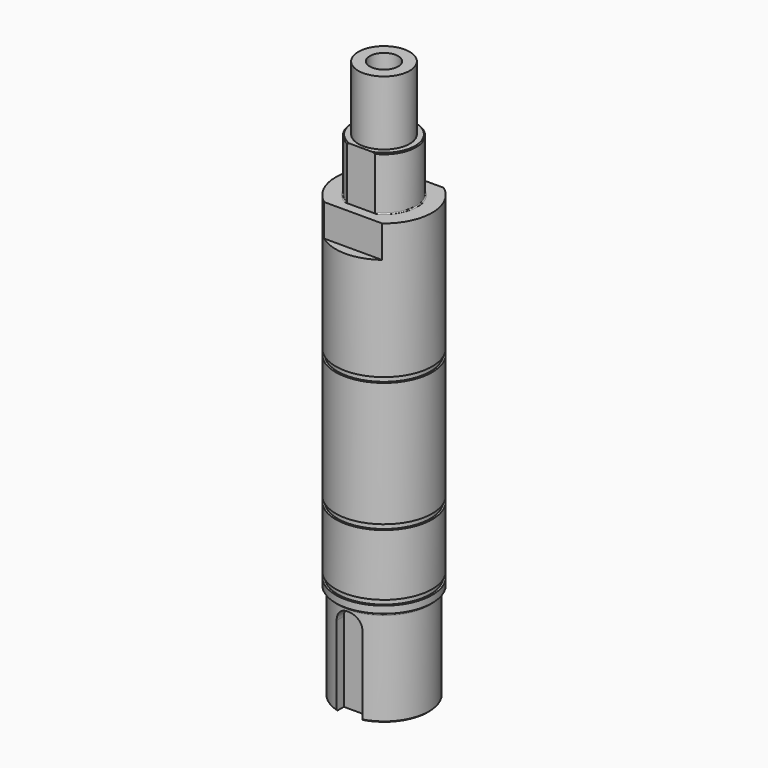
from build123d import *

# Parameters (mm, degrees)
F2_SIZE   = 0.29999
F4_DEPTH  = 28.8
F5_R      = 3.9999
F6_W      = 16.3141209632
F6_H      = 1.5053940788
F7_DEPTH  = 16.6
F8_W      = 11.3712083548
F8_H      = 5.6990628242
F9_DEPTH  = 10
F11_D     = 8.8
F11_DEPTH = 15
F11_TIP   = 2.6437867237


# Not quite as in the source:
# - a fillet or chamfer is up to 0.001 mm smaller than in the source, because OpenCascade refuses the exact size


with BuildPart() as f1:
    # F0 (on Front) → F1 (revolve)
    with BuildSketch(Plane.XZ):
        with BuildLine():
            Line((-14, 0), (0, 0))
            Line((0, 0), (0, 173.8))
            Line((0, 173.8), (-8, 173.8))
            Line((-8, 173.8), (-8, 153.8))
            Line((-8, 153.8), (-10, 153.8))
            Line((-10, 153.8), (-10, 137.5))
            ThreePointArc((-10, 137.5), (-10.0878679656, 137.2878679656), (-10.3, 137.2))
            Line((-10.3, 137.2), (-15, 137.2))
            Line((-15, 137.2), (-15, 137))
            Line((-15, 137), (-15, 136.8790119886))
            Line((-15, 136.8790119886), (-15, 95.1))
            Line((-15, 95.1), (-14.4, 95.1))
            Line((-14.4, 95.1), (-14.4, 93.5))
            Line((-14.4, 93.5), (-15, 93.5))
            Line((-15, 93.5), (-15, 54.8))
            Line((-15, 54.8), (-14.4, 54.8))
            Line((-14.4, 54.8), (-14.4, 53.2))
            Line((-14.4, 53.2), (-15, 53.2))
            Line((-15, 53.2), (-15, 34.1))
            Line((-15, 34.1), (-14.4, 34.1))
            Line((-14.4, 34.1), (-14.4, 32.5))
            Line((-14.4, 32.5), (-15, 32.5))
            Line((-15, 32.5), (-15, 30))
            Line((-15, 30), (-14.7, 30))
            ThreePointArc((-14.7, 30), (-14.2050252532, 29.7949747468), (-14, 29.3))
            Line((-14, 29.3), (-14, 0))
        make_face()
    revolve(axis=Axis((0, 0, 86.9), (0, 0, -1)))

    # F2 (size 0.3 in the source; OpenCascade refuses exactly that, so slightly less here)
    f2_edges = [f1.edges().sort_by_distance(p)[0] for p in [
        (15, 0, 30),
        (10, 0, 153.8),
        (14, 0, 0),
    ]]
    chamfer(f2_edges, length=F2_SIZE)

    # F3 (on face) → F4 (cut)
    with BuildSketch(Plane(origin=(0, 0, 0), x_dir=(1, 0, 0), z_dir=(0, 0, -1))):
        Polygon((4, 14), (0, 14), (-4, 14), (-4, 10.6), (0, 10.6), (4, 10.6), align=None)
    extrude(amount=-F4_DEPTH, mode=Mode.SUBTRACT)

    # F5 (radius 4 in the source; OpenCascade refuses exactly that, so slightly less here)
    f5_edges = [f1.edges().sort_by_distance(p)[0] for p in [
        (4, -12.008204, 28.8),
        (-4, -12.008204, 28.8),
    ]]
    fillet(f5_edges, radius=F5_R)

    # F6 (on face) → F7 (cut, through all)
    with BuildSketch(Plane.XY.offset(153.8)):
        with Locations((-8.1570604816, -9.7526970394)):
            Rectangle(F6_W, F6_H)
        with Locations((8.1570604816, -9.7526970394)):
            Rectangle(F6_W, F6_H)
        Polygon((-16.3141209632, 9), (0, 9), (16.3141209632, 9), (16.3141209632, 10.5053940788), (0, 10.5053940788), (-16.3141209632, 10.5053940788), align=None)
    extrude(amount=-F7_DEPTH, mode=Mode.SUBTRACT)

    # F8 (on face) → F9 (cut)
    with BuildSketch(Plane.XY.offset(137.2)):
        with Locations((5.6856041774, 14.8495314121)):
            Rectangle(F8_W, F8_H)
        with Locations((-5.6856041774, 14.8495314121)):
            Rectangle(F8_W, F8_H)
        Polygon((0, -17.6990628242), (11.3712083548, -17.6990628242), (11.3712083548, -12), (0, -12), (-11.3712083548, -12), (-11.3712083548, -17.6990628242), align=None)
    extrude(amount=-F9_DEPTH, mode=Mode.SUBTRACT)

    # F11
    with Locations(Plane.XY.offset(173.8)):
        with Locations((0, 0)):
            Hole(F11_D / 2, depth=F11_DEPTH)
            with Locations((0, 0, -(F11_DEPTH + F11_TIP / 2))):  # 118° drill point
                Cone(0, F11_D / 2, F11_TIP, mode=Mode.SUBTRACT)


solid = f1.part
